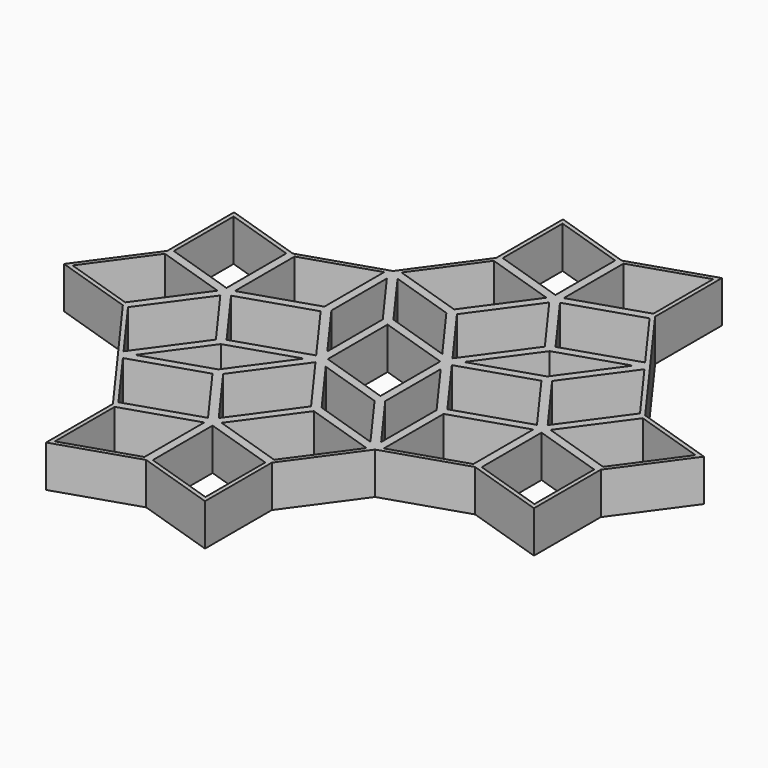
from build123d import *

# Parameters (mm, degrees)
F1_DEPTH = 3.175


# Not quite as in the source:
# - a feature names something its author has since deleted; it is built from what else it names


with BuildPart() as f1:
    # F0 (on Top) → F1 (new body)
    with BuildSketch(Plane.XY):
        Polygon((6.0392088785, 8.3122579143), (0, 6.35), (-6.0392088785, 8.3122579143), (-6.0392088785, 1.9622579143), (-9.7716452305, -3.175), (-3.7324363521, -5.1372579143), (0, -10.2745158286), (3.7324363521, -15.4117737428), (3.7324363521, -21.7617737428), (9.7716452305, -19.7995158286), (15.810854109, -21.7617737428), (15.810854109, -15.4117737428), (19.5432904611, -10.2745158286), (25.5824993395, -8.3122579143), (31.621708218, -10.2745158286), (31.621708218, -3.9245158286), (35.3541445701, 1.2127420857), (29.3149356916, 3.175), (25.5824993395, 8.3122579143), (21.8500629875, 13.4495158286), (21.8500629875, 19.7995158286), (15.810854109, 17.8372579143), (9.7716452305, 19.7995158286), (9.7716452305, 13.4495158286), align=None)
        Polygon((9.4541452305, -19.5688385759), (4.0499363521, -21.3247724831), (4.0499363521, -15.6424509955), (9.4541452305, -13.8865170883), align=None, mode=Mode.SUBTRACT)
        Polygon((0.5137257914, -10.4414354567), (5.9179346699, -8.6855015495), (9.2567076833, -13.2829899238), (3.8537105606, -15.0385301076), align=None, mode=Mode.SUBTRACT)
        Polygon((-9.2579194391, -3.0080803719), (-5.9179346699, 1.5890142791), (-0.5137257914, -0.1669196281), (-3.8537105606, -4.7640142791), align=None, mode=Mode.SUBTRACT)
        Polygon((-0.0007489063, -0.5411940443), (3.3399847692, -5.1372579143), (0, -9.7343525653), (-3.3399847692, -5.1372579143), align=None, mode=Mode.SUBTRACT)
        Polygon((3.9286621435, -5.4073395459), (8.9404194391, -3.7789208878), (5.842983087, -8.0421762826), (0.8312257914, -9.6705949407), align=None, mode=Mode.SUBTRACT)
        Polygon((9.7716452305, -3.7151632633), (13.1116299997, -8.3122579143), (9.7723941368, -12.9083217842), (6.4316604613, -8.3122579143), align=None, mode=Mode.SUBTRACT)
        Polygon((9.2579194391, -3.0080803719), (3.8537105606, -4.7640142791), (0.5149375472, -0.1665259048), (5.9179346699, 1.5890142791), align=None, mode=Mode.SUBTRACT)
        Polygon((10.0891452305, -2.9443227474), (10.0891452305, 2.7379987403), (15.493354109, 0.9820648331), (15.493354109, -4.7002566545), align=None, mode=Mode.SUBTRACT)
        Polygon((15.493354109, -15.6424509955), (15.493354109, -21.3247724831), (10.0891452305, -19.5688385759), (10.0891452305, -13.8865170883), align=None, mode=Mode.SUBTRACT)
        Polygon((13.6253557912, -8.6855015495), (19.0295646696, -10.4414354567), (15.6895799004, -15.0385301076), (10.285371022, -13.2825962005), align=None, mode=Mode.SUBTRACT)
        Polygon((15.6146283176, -5.4073395459), (18.7120646696, -9.6705949407), (13.700307374, -8.0421762826), (10.602871022, -3.7789208878), align=None, mode=Mode.SUBTRACT)
        Polygon((19.2257904611, -9.2973513055), (16.128354109, -5.0340959107), (16.128354109, 0.2355775627), (19.2257904611, -4.0276778321), align=None, mode=Mode.SUBTRACT)
        Polygon((19.8607904611, -9.8375145688), (19.8607904611, -4.1551930812), (25.2649993395, -2.399259174), (25.2649993395, -8.0815806616), align=None, mode=Mode.SUBTRACT)
        Polygon((31.304208218, -9.8375145688), (25.8999993395, -8.0815806616), (25.8999993395, -2.399259174), (31.304208218, -4.1551930812), align=None, mode=Mode.SUBTRACT)
        Polygon((-5.7217088785, 7.8752566545), (-0.3175, 6.1193227474), (-0.3175, 0.4370012597), (-5.7217088785, 2.1929351669), align=None, mode=Mode.SUBTRACT)
        Polygon((5.7217088785, 7.8752566545), (5.7217088785, 2.1929351669), (0.3175, 0.4370012597), (0.3175, 6.1193227474), align=None, mode=Mode.SUBTRACT)
        Polygon((6.3567088785, 2.0654199178), (6.3567088785, 7.3350933912), (9.4541452305, 3.0718379964), (9.4541452305, -2.1978354769), align=None, mode=Mode.SUBTRACT)
        Polygon((9.967871022, 3.4450816317), (6.8704346699, 7.7083370264), (11.8821919655, 6.0799183683), (14.9796283176, 1.8166629736), align=None, mode=Mode.SUBTRACT)
        Polygon((6.5529346699, 8.4791775424), (9.8929194391, 13.0762721934), (15.2971283176, 11.3203382862), (11.9571435484, 6.7232436352), align=None, mode=Mode.SUBTRACT)
        Polygon((25.0675617923, -1.7957320095), (19.6645646696, -3.5512721934), (16.3245799004, 1.0458224576), (21.7287887789, 2.8017563648), align=None, mode=Mode.SUBTRACT)
        Polygon((15.810854109, 1.752905349), (12.4708693398, 6.35), (15.8101052028, 10.94606387), (19.1508388782, 6.35), align=None, mode=Mode.SUBTRACT)
        Polygon((21.6538371961, 3.4450816317), (16.6420799004, 1.8166629736), (19.7395162525, 6.0799183683), (24.7512735481, 7.7083370264), align=None, mode=Mode.SUBTRACT)
        Polygon((25.5832482458, -1.42106387), (22.2425145703, 3.175), (25.5824993395, 7.772094651), (28.9224841087, 3.175), align=None, mode=Mode.SUBTRACT)
        Polygon((29.4362099002, 2.8017563648), (34.8404187786, 1.0458224576), (31.5004340094, -3.5512721934), (26.096225131, -1.7953382862), align=None, mode=Mode.SUBTRACT)
        Polygon((21.7287887789, 13.0762721934), (25.0687735481, 8.4791775424), (19.6645646696, 6.7232436352), (16.3257916562, 11.3207320095), align=None, mode=Mode.SUBTRACT)
        Polygon((10.0891452305, 13.6801930812), (10.0891452305, 19.3625145688), (15.493354109, 17.6065806616), (15.493354109, 11.924259174), align=None, mode=Mode.SUBTRACT)
        Polygon((16.128354109, 17.6065806616), (21.5325629875, 19.3625145688), (21.5325629875, 13.6801930812), (16.128354109, 11.924259174), align=None, mode=Mode.SUBTRACT)
    extrude(amount=F1_DEPTH)


solid = f1.part
